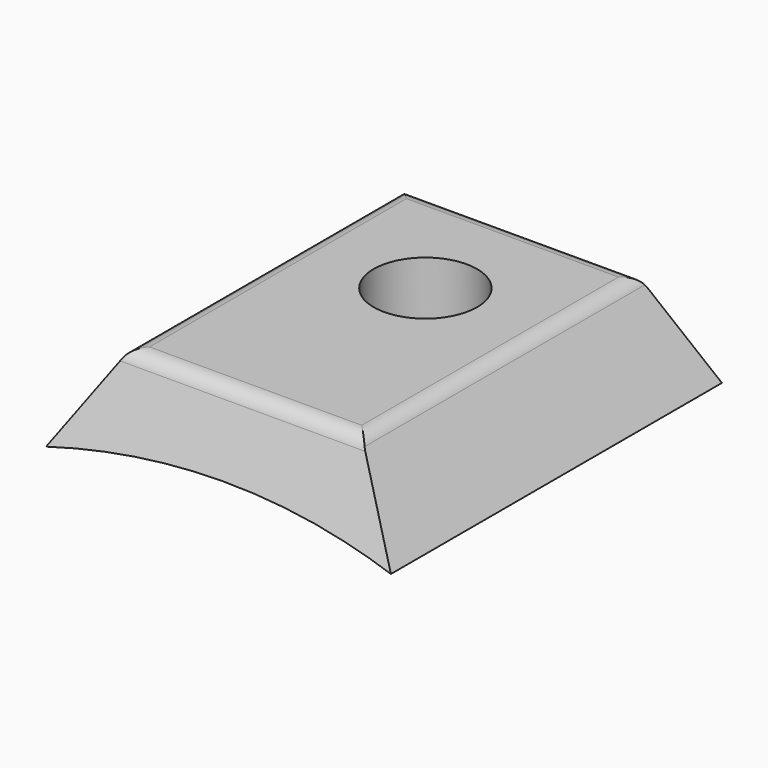
from build123d import *

# Parameters (mm, degrees)
F1_DEPTH = 60
F3_DEPTH = 75
F4_R     = 15
F5_DEPTH = 25


# Not quite as in the source:
# - a feature names something its author has since deleted; it is built from what else it names


with BuildPart() as f1:
    # F0 (on Front) → F1 (new body, symmetric)
    with BuildSketch(Plane.XZ):
        with BuildLine():
            ThreePointArc((-50, 196.9523800313), (0, 203.2), (50, 196.9523800313))
            Line((50, 196.9523800313), (35, 220.857542129))
            ThreePointArc((35, 220.857542129), (33.1846822218, 222.5753691641), (30.7647349749, 223.2))
            Line((30.7647349749, 223.2), (-30.7647349749, 223.2))
            ThreePointArc((-30.7647349749, 223.2), (-33.1846822218, 222.5753691641), (-35, 220.857542129))
            Line((-35, 220.857542129), (-50, 196.9523800313))
        make_face()
    extrude(amount=F1_DEPTH, both=True)

    # F2 (on Right) → F3 (cut, symmetric)
    with BuildSketch(Plane.YZ):
        with BuildLine():
            Line((60, 223.2), (46.5543481195, 223.2))
            ThreePointArc((46.5543481195, 223.2), (49.3915485081, 222.3170734697), (51.2267330988, 219.980117582))
            Line((51.2267330988, 219.980117582), (60, 196.9523800313))
            Line((60, 196.9523800313), (60, 223.2))
        make_face()
        with BuildLine():
            ThreePointArc((-51.2267330988, 219.980117582), (-49.3915485081, 222.3170734697), (-46.5543481195, 223.2))
            Line((-46.5543481195, 223.2), (-60, 223.2))
            Line((-60, 223.2), (-60, 196.9523800313))
            Line((-60, 196.9523800313), (-51.2267330988, 219.980117582))
        make_face()
    extrude(amount=F3_DEPTH, both=True, mode=Mode.SUBTRACT)

    # F4 (on face) → F5 (cut)
    with BuildSketch(Plane.XY.offset(223.2)):
        with Locations((0, 15)):
            Circle(F4_R)
    extrude(amount=-F5_DEPTH, mode=Mode.SUBTRACT)


solid = f1.part
